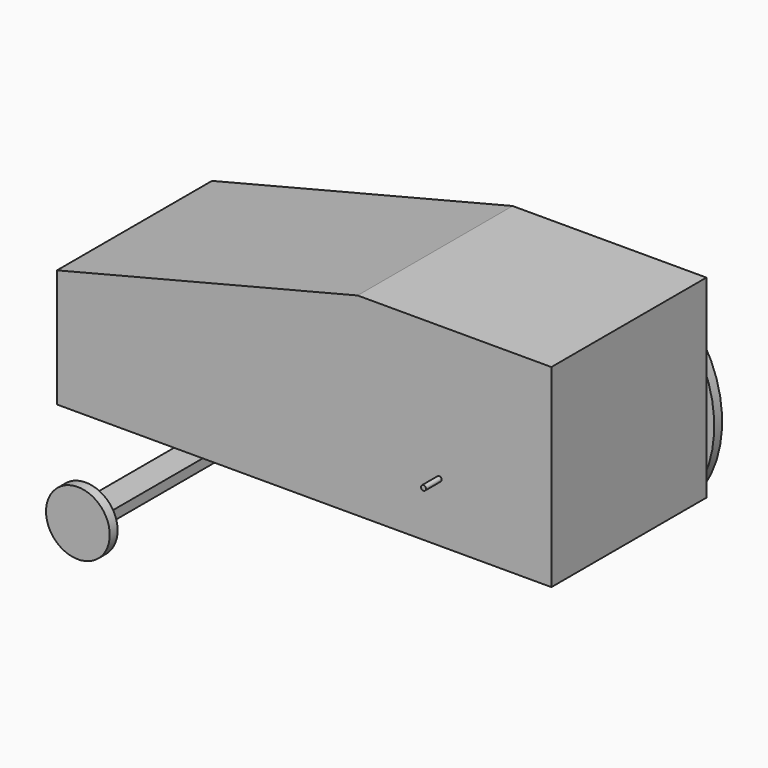
from build123d import *

# Parameters (mm, degrees)
F1_DEPTH  = 500
F2_W      = 73.9309489727
F2_H      = 500
F2_H_2    = 305.1662445068
F2_H_3    = 304.9542307854
F3_DEPTH  = 25.4
F4_R      = 5.11898469
F5_DEPTH  = 50.8
F6_R      = 82.2041903744
F6_R_2    = 5.11898469
F7_DEPTH  = 25.4
F8_R      = 5.8344538593
F9_DEPTH  = 50.8
F10_R     = 76.2
F11_DEPTH = 25.4
F12_R     = 6.35
F13_DEPTH = 50.8
F14_R     = 304.8
F14_R_2   = 6.35
F15_DEPTH = 25.4
F16_R     = 6.35
F17_DEPTH = 50.8


with BuildPart() as f1:
    # F0 (on Front) → F1 (new body)
    with BuildSketch(Plane.XZ):
        Polygon((-775.8201853523, 304.8), (-775.8201853523, 0), (500, 0), (500, 500), (0, 500), align=None)
    extrude(amount=F1_DEPTH)

    # F2 (on face) → F3 (join)
    with BuildSketch(Plane(origin=(0, 0, 0), x_dir=(1, 0, 0), z_dir=(0, 0, -1))):
        with Locations((-436.6519004107, 250)):
            Rectangle(F2_W, F2_H)
        with Locations((-436.6519004107, 652.5831222534)):
            Rectangle(F2_W, F2_H_2)
        with Locations((-436.6519004107, -152.4771153927)):
            Rectangle(F2_W, F2_H_3)
    extrude(amount=F3_DEPTH)

    # F4 (on face) → F5 (join)
    with BuildSketch(Plane.XZ.offset(805.1662445068)):
        with Locations((-437.0749592781, -14.6776270121)):
            Circle(F4_R)
    extrude(amount=F5_DEPTH)

    # F6 (on face) → F7 (join)
    with BuildSketch(Plane.XZ.offset(855.9662445068)):
        with Locations((-437.0749592781, -14.6776270121)):
            Circle(F6_R)
        with Locations((-437.0749592781, -14.6776270121)):
            Circle(F6_R_2, mode=Mode.SUBTRACT)
    extrude(amount=-F7_DEPTH)

    # F8 (on face) → F9 (join)
    with BuildSketch(Plane(origin=(0, 304.9542307854, 0), x_dir=(-1, 0, 0), z_dir=(0, 1, 0))):
        with Locations((435.6042742729, -14.3710989505)):
            Circle(F8_R)
    extrude(amount=F9_DEPTH)

    # F10 (on face) → F11 (join)
    with BuildSketch(Plane(origin=(0, 355.7542307854, 0), x_dir=(-1, 0, 0), z_dir=(0, 1, 0))):
        with Locations((435.6042742729, -14.3710989505)):
            Circle(F10_R)
    extrude(amount=-F11_DEPTH)

    # F12 (on face) → F13 (join)
    with BuildSketch(Plane.XZ):
        with Locations((195.2, 152.4)):
            Circle(F12_R)
    extrude(amount=-F13_DEPTH)

    # F14 (on face) → F15 (join)
    with BuildSketch(Plane(origin=(0, 50.8, 0), x_dir=(-1, 0, 0), z_dir=(0, 1, 0))):
        with Locations((-195.2, 152.4)):
            Circle(F14_R)
        with Locations((-195.2, 152.4)):
            Circle(F14_R_2, mode=Mode.SUBTRACT)
    extrude(amount=-F15_DEPTH)

    # F16 (on face) → F17 (join)
    with BuildSketch(Plane.XZ.offset(500)):
        with Locations((210.5554491282, 151.9356071949)):
            Circle(F16_R)
    extrude(amount=F17_DEPTH)


solid = f1.part
